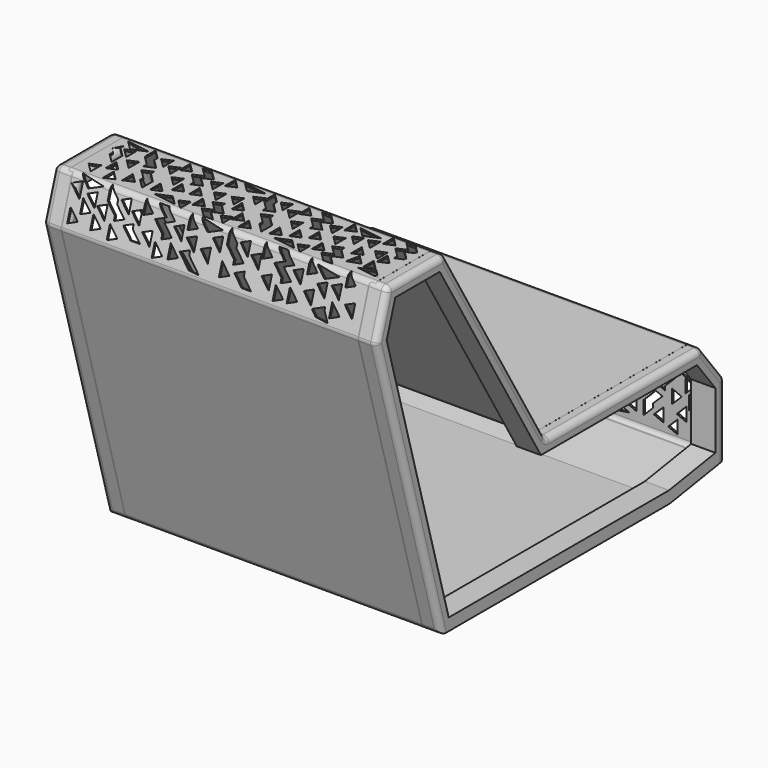
from build123d import *

# Parameters (mm, degrees)
F1_DEPTH  = 50.8
F2_R      = 12.7
F6_DEPTH  = 322.834
F9_DEPTH  = 25.4
F10_DEPTH = 25.4
F13_DEPTH = 25.4


with BuildPart() as f1:
    # F0 (on Right) → F1 (new body)
    with BuildSketch(Plane.YZ):
        Polygon((408.05088859, 0), (0, 0), (-265.7088614251, 447.3610464164), (-415.7088614251, 447.3610464164), (-446.1864444173, 352.1186349866), (-275.8783534847, -252.6389535836), (324.1216465153, -252.6389535836), (469.3139055241, -229.0369708183), (469.3139055241, -79.0369708183), align=None)
        Polygon((-256.6433629502, -227.2389464719), (-419.6670120859, 351.6518648302), (-397.1680678867, 421.9610393047), (-280.1650366436, 421.9610393047), (-14.4561752185, -25.4000071117), (395.6020354119, -25.4000071117), (443.9138984125, -87.7283660016), (443.9138984125, -207.4325008904), (322.0706361109, -227.2389464719), align=None, mode=Mode.SUBTRACT)
    extrude(amount=F1_DEPTH)

    # F2
    f2_edges = [f1.edges().sort_by_distance(p)[0] for p in [
        (25.4, -265.708861, 447.361046),
        (25.4, -415.708861, 447.361046),
        (0, -340.708861, 447.361046),
        (50.8, -340.708861, 447.361046),
        (25.4, 0, 0),
        (0, -132.854431, 223.680523),
        (50.8, -132.854431, 223.680523),
        (25.4, 408.050889, 0),
        (0, 204.025444, 0),
        (50.8, 204.025444, 0),
        (25.4, 469.313906, -79.036971),
        (0, 438.682397, -39.518485),
        (50.8, 438.682397, -39.518485),
        (25.4, 469.313906, -229.036971),
        (0, 469.313906, -154.036971),
        (50.8, 469.313906, -154.036971),
        (25.4, -446.186444, 352.118635),
        (25.4, -275.878353, -252.638954),
        (0, -361.032399, 49.739841),
        (50.8, -361.032399, 49.739841),
        (0, -430.947653, 399.739841),
        (50.8, -430.947653, 399.739841),
    ]]
    fillet(f2_edges, radius=F2_R)


with BuildPart() as f4_1:
    # F4: instance of F1
    add(f1.part.mirror(Plane.YZ.offset(-300)))


with BuildPart() as f6:
    # F5 (on offset) → F6 (new body, symmetric)
    with BuildSketch(Plane.YZ.offset(-300)):
        with BuildLine():
            Line((-272.8356088733, 447.4316021146), (-406.3371291142, 447.4316021146))
            ThreePointArc((-406.3371291142, 447.4316021146), (-413.8248759846, 444.9894599223), (-418.4329153658, 438.6022551546))
            Line((-418.4329153658, 438.6022551546), (-444.9211800784, 355.8264587119))
            ThreePointArc((-444.9211800784, 355.8264587119), (-445.5234270705, 352.1793045345), (-445.0499009192, 348.513215608))
            Line((-445.0499009192, 348.513215608), (-278.3840298653, -243.3109879494))
            ThreePointArc((-278.3840298653, -243.3109879494), (-273.8266312953, -249.992895251), (-266.1595227729, -252.5683978854))
            Line((-266.1595227729, -252.5683978854), (-262.5830273378, -252.5683978854))
            Line((-262.5830273378, -252.5683978854), (324.2229846526, -252.5683978854))
            Line((324.2229846526, -252.5683978854), (456.7152436615, -231.0308859339))
            Line((456.7152436615, -231.0308859339), (458.7529669103, -230.699640251))
            ThreePointArc((458.7529669103, -230.699640251), (466.3891540719, -226.3925157803), (469.4152436615, -218.1641831807))
            Line((469.4152436615, -218.1641831807), (469.4152436615, -83.312111495))
            ThreePointArc((469.4152436615, -83.312111495), (468.7312482019, -79.2004652452), (466.7529389554, -75.5317083444))
            Line((466.7529389554, -75.5317083444), (411.9654971749, -4.8490411512))
            ThreePointArc((411.9654971749, -4.8490411512), (407.5170272293, -1.2254730634), (401.927801881, 0.0705556982))
            Line((401.927801881, 0.0705556982), (7.3294237228, 0.0705556982))
            ThreePointArc((7.3294237228, 0.0705556982), (1.0475059475, 1.7330057407), (-3.5897859266, 6.2851211999))
            Line((-3.5897859266, 6.2851211999), (-261.9163992238, 441.2170366128))
            ThreePointArc((-261.9163992238, 441.2170366128), (-266.5536910979, 445.769152072), (-272.8356088733, 447.4316021146))
        make_face()
        with BuildLine():
            ThreePointArc((-414.8041674125, 437.4410553777), (-411.5785444469, 441.9120923374), (-406.3371291142, 443.6215894334))
            Line((-406.3371291142, 443.6215894334), (-272.8356088733, 443.6215894334))
            ThreePointArc((-272.8356088733, 443.6215894334), (-268.4382727031, 442.4578760637), (-265.1921730216, 439.2713997876))
            Line((-265.1921730216, 439.2713997876), (-6.8655597245, 4.3394843746))
            ThreePointArc((-6.8655597245, 4.3394843746), (-0.8370756577, -1.5782702677), (7.3294237228, -3.739456983))
            Line((7.3294237228, -3.739456983), (401.927801881, -3.739456983))
            ThreePointArc((401.927801881, -3.739456983), (405.8402540439, -4.646675822), (408.954178564, -7.1831698652))
            Line((408.954178564, -7.1831698652), (463.7416203444, -77.8658370584))
            ThreePointArc((463.7416203444, -77.8658370584), (465.1264348416, -80.4339632257), (465.6052309803, -83.312111495))
            Line((465.6052309803, -83.312111495), (465.6052309803, -218.1641831807))
            ThreePointArc((465.6052309803, -218.1641831807), (463.4869712893, -223.9240077843), (458.1416479009, -226.938990613))
            Line((458.1416479009, -226.938990613), (456.1039246521, -227.270236296))
            Line((456.1039246521, -227.270236296), (323.9153321541, -248.7583852043))
            Line((323.9153321541, -248.7583852043), (-262.5830273378, -248.7583852043))
            Line((-262.5830273378, -248.7583852043), (-266.1595227729, -248.7583852043))
            ThreePointArc((-266.1595227729, -248.7583852043), (-271.5264910828, -246.9555359319), (-274.7166655312, -242.2782074927))
            Line((-274.7166655312, -242.2782074927), (-441.3825365851, 349.5459960647))
            ThreePointArc((-441.3825365851, 349.5459960647), (-441.7140044182, 352.1122546526), (-441.2924321251, 354.665258935))
            Line((-441.2924321251, 354.665258935), (-414.8041674125, 437.4410553777))
        make_face(mode=Mode.SUBTRACT)
    extrude(amount=F6_DEPTH, both=True)

    # F8 (on face) → F9 (cut)
    with BuildSketch(Plane(origin=(0, -506.8810328427, 162.2019908326), x_dir=(1, 0, 0), z_dir=(0, -0.9524241143, 0.3047758299))):
        Polygon((-610.2134572743, 280.1658902577), (-587.9954886436, 258.1666408395), (-587.9954886436, 289.7434858457), align=None)
        Polygon((-553.3538012807, 290.2071253475), (-584.2335065195, 290.2071253475), (-575.091958046, 281.1555685521), align=None)
        Polygon((-545.7693254662, 293.3652272206), (-595.091958046, 300.9586835748), (-584.2335065195, 290.2071253475), (-553.3538012807, 290.2071253475), align=None)
        Polygon((-574.9599039268, 272.0962909685), (-554.9599039268, 252.2931759458), (-554.9599039268, 280.7177772503), align=None)
        Polygon((-561.2534010124, 243.4772804856), (-581.2534010124, 263.2803955084), (-581.2534010124, 234.8557942038), align=None)
        Polygon((-602.6199054718, 241.1658143859), (-602.6199054718, 212.7412130814), (-582.6199054718, 221.3626993632), align=None)
        Polygon((-554.9599039268, 243.671689664), (-554.9599039268, 215.2470883594), (-534.9599039268, 223.8685746412), align=None)
        Polygon((-550.9002315712, 258.1129518972), (-530.9002315712, 238.3098368745), (-530.9002315712, 266.734438179), align=None)
        Polygon((-521.3424320719, 290.2071253475), (-532.2008835983, 290.2071253475), (-532.2008835983, 272.5340822703), (-512.2008835983, 252.7309672475), (-512.2008835983, 244.1094809657), (-492.2008835983, 252.7309672475), (-512.2008835983, 272.5340822703), (-512.2008835983, 281.1555685521), align=None)
        Polygon((-532.2008835983, 300.9586835748), (-532.2008835983, 290.2071253475), (-521.3424320719, 290.2071253475), align=None)
        Polygon((-485.7396268845, 290.2071253475), (-487.70695417, 290.2071253475), (-505.7396268845, 282.4337033258), (-485.7396268845, 262.6305883031), align=None)
        Polygon((-498.8226485252, 217.7414104819), (-518.8226485252, 237.5445255047), (-518.8226485252, 209.1199242001), align=None)
        Polygon((-472.2404265404, 222.5241366963), (-452.2404265404, 222.5241366963), (-472.2404265404, 242.3272517191), (-472.2404265404, 250.9487380009), (-492.2404265404, 242.3272517191), align=None)
        Polygon((-480.7777786255, 270.2546862589), (-460.7777786255, 250.4515712361), (-460.7777786255, 278.8761725407), align=None)
        Polygon((-449.0202209381, 290.2071253475), (-458.018758297, 290.2071253475), (-458.018758297, 270.6924775606), (-438.018758297, 279.3139638424), align=None)
        Polygon((-458.018758297, 299.1170788652), (-458.018758297, 290.2071253475), (-449.0202209381, 290.2071253475), align=None)
        Polygon((-431.9680453543, 299.385476847), (-422.6984415682, 290.2071253475), (-403.0085313252, 290.2071253475), (-412.2482537937, 299.3558896886), align=None)
        Polygon((-403.0085313252, 290.2071253475), (-422.6984415682, 290.2071253475), (-412.3803079128, 279.9905659676), (-432.3803079128, 271.3690796858), (-412.3803079128, 251.5659646631), (-412.2482537937, 242.5066870795), (-392.2482537937, 251.1281733613), (-412.2482537937, 270.9312883841), (-392.2482537937, 279.5527746659), align=None)
        Polygon((-432.3803079128, 223.1413633585), (-432.3803079128, 251.5659646631), (-452.3803079128, 242.9444783813), align=None)
        Polygon((-403.8098454475, 215.9172997356), (-423.8098454475, 235.7204147583), (-423.8098454475, 207.2958134538), align=None)
        Polygon((-392.2482537937, 242.5066870795), (-392.2482537937, 214.082085775), (-372.2482537937, 222.7035720568), align=None)
        Polygon((-392.2482537937, 270.9312883841), (-372.2482537937, 251.1281733613), (-372.2482537937, 279.5527746659), align=None)
        Polygon((-353.3391356283, 290.2071253475), (-364.628246994, 290.2071253475), (-364.628246994, 272.9605025869), (-344.628246994, 281.5819888687), align=None)
        Polygon((-364.628246994, 301.3851038914), (-364.628246994, 290.2071253475), (-353.3391356283, 290.2071253475), align=None)
        Polygon((-344.628246994, 301.3851038914), (-333.3391356283, 290.2071253475), (-303.9141783387, 290.2071253475), (-295.3056144142, 293.7916475372), align=None)
        Polygon((-303.9141783387, 290.2071253475), (-333.3391356283, 290.2071253475), (-324.628246994, 281.5819888687), align=None)
        Polygon((-343.1586944771, 240.5479399776), (-343.1586944771, 268.9725412821), (-363.1586944771, 260.3510550003), align=None)
        Polygon((-351.315243187, 233.4173643909), (-351.4472973061, 242.4766419744), (-371.4472973061, 233.8551556926), (-346.7147119375, 209.3660440495), (-324.8525857925, 207.1910202503), align=None)
        Polygon((-331.7133914852, 250.4200275026), (-311.7133914852, 230.6169124798), (-311.7133914852, 259.0415137844), align=None)
        Polygon((-312.1250509644, 275.4354114614), (-292.1250509644, 255.6322964386), (-292.1250509644, 284.0568977432), align=None)
        Polygon((-270.4480611807, 290.2071253475), (-281.7371725464, 290.2071253475), (-281.7371725464, 272.9605025869), (-261.7371725464, 253.1573875641), (-261.7371725464, 244.5359012824), (-241.7371725464, 253.1573875641), (-261.7371725464, 272.9605025869), (-261.7371725464, 281.5819888687), align=None)
        Polygon((-281.7371725464, 301.3851038914), (-281.7371725464, 290.2071253475), (-270.4480611807, 290.2071253475), align=None)
        Polygon((-284.7306370163, 244.4622198544), (-284.7306370163, 216.0376185498), (-264.7306370163, 224.6591048316), align=None)
        Polygon((-236.1780321312, 212.2973443464), (-216.1780321312, 212.2973443464), (-236.1780321312, 232.1004593692), (-236.1780321312, 240.721945651), (-256.1780321312, 232.1004593692), align=None)
        Polygon((-236.1780619335, 264.8613008217), (-236.1780619335, 290.2071253475), (-243.3201640681, 290.2071253475), (-256.1780619335, 284.6644158445), align=None)
        Polygon((-243.3201640681, 290.2071253475), (-236.1780619335, 290.2071253475), (-236.1780619335, 293.2859021263), align=None)
        Polygon((-207.555047245, 290.2071253475), (-198.1258500469, 290.2071253475), (-207.555047245, 299.5434991818), align=None)
        Polygon((-187.555047245, 279.7403841591), (-198.1258500469, 290.2071253475), (-207.555047245, 290.2071253475), (-207.555047245, 271.1188978773), align=None)
        Polygon((-230.3140675735, 270.6811065755), (-210.3140675735, 250.8779915528), (-210.3140675735, 279.3025928573), align=None)
        Polygon((-181.9165968609, 223.5677836751), (-181.9165968609, 251.9923849797), (-201.9165968609, 243.3708986979), align=None)
        Polygon((-150.3972542, 218.5057593321), (-170.3972542, 238.3088743549), (-170.3972542, 209.8842730503), align=None)
        Polygon((-141.7845427418, 279.9791949825), (-152.114160434, 290.2071253475), (-171.804070677, 290.2071253475), (-161.9165968609, 280.4169862842), (-181.9165968609, 271.7955000024), (-161.9165968609, 251.9923849797), (-161.7845427418, 242.9331073961), (-141.7845427418, 251.5545936779), (-161.7845427418, 271.3577087007), align=None)
        Polygon((-171.804070677, 290.2071253475), (-152.114160434, 290.2071253475), (-161.7845427418, 299.7823100052), (-181.5043343023, 299.8118971637), align=None)
        Polygon((-113.2840113342, 290.2071253475), (-102.2302799566, 290.2071253475), (-113.2840113342, 301.1520410425), align=None)
        Polygon((-93.2840113342, 281.3489260197), (-102.2302799566, 290.2071253475), (-113.2840113342, 290.2071253475), (-113.2840113342, 272.7274397379), align=None)
        Polygon((-141.7845427418, 271.3577087007), (-121.7845427418, 251.5545936779), (-121.7845427418, 279.9791949825), align=None)
        Polygon((-93.2840113342, 224.4997234106), (-93.2840113342, 252.9243247152), (-113.2840113342, 244.3028384334), align=None)
        Polygon((-141.7845427418, 242.9331073961), (-141.7845427418, 214.5085060916), (-121.7845427418, 223.1299923734), align=None)
        Polygon((-64.8736751787, 225.3813321149), (-64.9616606534, 231.4173788786), (-90.336183123, 220.4790740097), (-80.0273045897, 209.706902504), (-54.0199615061, 206.7942172289), align=None)
        Polygon((-53.1519572151, 243.8650471316), (-53.1519572151, 215.4404458271), (-33.1519572151, 224.0619321089), align=None)
        Polygon((-7.5135068309, 226.7677186346), (-7.5135068309, 255.1923199391), (-27.5135068309, 246.5708336573), align=None)
        Polygon((-60.820243777, 269.5832101332), (-40.820243777, 249.7800951104), (-40.820243777, 278.204696415), align=None)
        Polygon((-89.8417569411, 263.7192157732), (-69.8417569411, 243.9161007505), (-69.8417569411, 272.340702055), align=None)
        Polygon((-48.0119017971, 287.9891266804), (-62.4187184316, 290.2071253475), (-91.9056332358, 290.2071253475), (-77.3345343769, 275.7794680119), align=None)
        Polygon((-91.9056332358, 290.2071253475), (-62.4187184316, 290.2071253475), (-97.3345343769, 295.5825830346), align=None)
        Polygon((-33.1519572151, 290.2071253475), (-20.4910109151, 290.2071253475), (-33.1519572151, 302.7434341412), align=None)
        Polygon((-13.1519572151, 282.9403191185), (-20.4910109151, 290.2071253475), (-33.1519572151, 290.2071253475), (-33.1519572151, 274.3188328367), align=None)
    extrude(amount=-F9_DEPTH, mode=Mode.SUBTRACT)

    # F7 (on face) → F10 (cut)
    with BuildSketch(Plane.XY.offset(447.4316021146)):
        Polygon((-558.2723617554, -283.5318148136), (-607.5949943352, -275.9383584594), (-587.5949943352, -295.7414734821), align=None)
        Polygon((-602.6913714409, -330.5999256248), (-582.6913714409, -350.4030406475), (-582.6913714409, -321.978439343), (-602.6913714409, -302.1753243202), (-602.6913714409, -293.5538380384), (-612.6913714409, -312.0768818316), (-602.6913714409, -321.978439343), align=None)
        Polygon((-595.1479458809, -301.6980014795), (-575.1479458809, -321.5011165023), (-575.1479458809, -293.0765151978), align=None)
        Polygon((-608.7343287468, -378.1811335678), (-588.7343287468, -397.9842485905), (-588.7343287468, -369.559647286), align=None)
        Polygon((-576.9602847099, -344.9864812726), (-576.9602847099, -373.4110825772), (-556.9602847099, -364.7895962954), align=None)
        Polygon((-538.9182567596, -394.1856687169), (-558.9182567596, -374.3825536942), (-558.9182567596, -402.8071549987), align=None)
        Polygon((-567.4963188171, -329.8447750563), (-547.4963188171, -349.647890079), (-547.4963188171, -321.2232887745), align=None)
        Polygon((-532.3889255524, -292.638723896), (-552.3889255524, -272.8356088733), (-552.3889255524, -301.2602101778), (-532.3889255524, -321.0633252005), (-532.3889255524, -329.6848114823), (-512.3889255524, -321.0633252005), (-532.3889255524, -301.2602101778), align=None)
        Polygon((-525.9276688385, -291.3605891222), (-505.9276688385, -311.163704145), (-505.9276688385, -282.7391028404), align=None)
        Polygon((-500.9658205795, -303.5396061892), (-480.9658205795, -323.3427212119), (-480.9658205795, -294.9181199074), align=None)
        Polygon((-506.8297851372, -370.5448547), (-486.8297851372, -390.3479697228), (-486.8297851372, -361.9233684183), (-506.8297851372, -342.1202533955), (-506.8297851372, -333.4987671137), (-526.8297851372, -342.1202533955), (-506.8297851372, -361.9233684183), align=None)
        Polygon((-508.7803411484, -381.5211420159), (-528.7803411484, -361.7180269932), (-528.7803411484, -390.1426282977), align=None)
        Polygon((-452.5683498669, -350.6529290895), (-452.5683498669, -322.228327785), (-472.5683498669, -330.8498140668), align=None)
        Polygon((-452.5683498669, -379.0775303941), (-472.5683498669, -359.2744153713), (-472.5683498669, -387.6990166759), align=None)
        Polygon((-458.206800251, -294.4803286056), (-478.206800251, -274.6772135829), (-478.206800251, -303.1018148874), align=None)
        Polygon((-432.5683498669, -322.228327785), (-432.4362957478, -331.2876053685), (-412.4362957478, -322.6661190868), (-432.4362957478, -302.863004064), (-412.4362957478, -294.2415177822), (-432.4362957478, -274.4384027595), (-452.1560873083, -274.408815601), (-432.5683498669, -293.8037264805), (-452.5683498669, -302.4252127623), align=None)
        Polygon((-423.9978874016, -357.8769927125), (-443.9978874016, -338.0738776898), (-443.9978874016, -366.4984789943), align=None)
        Polygon((-457.7084052849, -394.7770086383), (-408.3857727051, -402.3704649926), (-428.3857727051, -382.5673499698), align=None)
        Polygon((-412.4362957478, -388.1368079776), (-394.0550248057, -406.3371291142), (-392.4362957478, -406.3371291142), (-392.4362957478, -379.5153216958), align=None)
        Polygon((-412.4362957478, -331.2876053685), (-412.4362957478, -359.7122066731), (-392.4362957478, -351.0907203913), align=None)
        Polygon((-412.4362957478, -302.863004064), (-392.4362957478, -322.6661190868), (-392.4362957478, -294.2415177822), align=None)
        Polygon((-384.3856291088, -272.8356088733), (-384.8162889481, -272.8356088733), (-384.8162889481, -300.8337898612), (-364.8162889481, -292.2123035794), align=None)
        Polygon((-364.8162889481, -349.0615061885), (-364.8162889481, -320.6369048839), (-384.8162889481, -329.2583911657), align=None)
        Polygon((-364.8162889481, -377.486107493), (-384.8162889481, -357.6829924703), (-384.8162889481, -386.1075937748), align=None)
        Polygon((-344.6842348289, -358.120783772), (-344.8162889481, -349.0615061885), (-364.8162889481, -357.6829924703), (-344.8162889481, -377.486107493), (-364.8162889481, -386.1075937748), (-344.8162889481, -405.9107087975), (-325.0964973875, -405.940295956), (-344.6842348289, -386.5453850765), (-324.6842348289, -377.9238987948), align=None)
        Polygon((-362.0465130225, -272.8356088733), (-364.3856291088, -272.8356088733), (-344.8162889481, -292.2123035794), (-315.4936563683, -280.0026449109), align=None)
        Polygon((-324.6842348289, -301.2715811629), (-304.6842348289, -321.0746961857), (-304.6842348289, -292.6500948811), align=None)
        Polygon((-324.6842348289, -329.6961824675), (-324.6842348289, -358.120783772), (-304.6842348289, -349.4992974902), align=None)
        Polygon((-324.6842348289, -386.5453850765), (-304.6957188658, -406.3371291142), (-304.6842348289, -406.3371291142), (-304.6842348289, -377.9238987948), align=None)
        Polygon((-281.9252145004, -377.486107493), (-301.9252145004, -357.6829924703), (-301.9252145004, -386.1075937748), align=None)
        Polygon((-256.9633960438, -391.4694465643), (-276.9633960438, -371.6663315415), (-276.9633960438, -400.0909328461), align=None)
        Polygon((-256.3660740852, -370.1184343834), (-236.3660740852, -389.9215494062), (-236.3660740852, -361.4969481016), (-256.3660740852, -341.6938330789), (-256.3660740852, -333.0723467971), (-276.3660740852, -341.6938330789), (-256.3660740852, -361.4969481016), align=None)
        Polygon((-301.4945546612, -272.8356088733), (-301.9252145004, -272.8356088733), (-301.9252145004, -300.8337898612), (-281.9252145004, -320.6369048839), (-281.9252145004, -329.2583911657), (-261.9252145004, -320.6369048839), (-281.9252145004, -300.8337898612), (-281.9252145004, -292.2123035794), align=None)
        Polygon((-276.3661038876, -289.1298766036), (-256.3661038876, -308.9329916263), (-256.3661038876, -280.5083903218), align=None)
        Polygon((-250.5021095276, -303.1131858725), (-230.5021095276, -322.9163008953), (-230.5021095276, -294.4916995908), align=None)
        Polygon((-207.7430891991, -294.053908289), (-227.7430891991, -274.2507932663), (-227.7430891991, -302.6753945708), align=None)
        Polygon((-202.1046388149, -350.2265087729), (-202.1046388149, -321.8019074684), (-222.1046388149, -330.4233937502), align=None)
        Polygon((-202.1046388149, -378.6511100775), (-222.1046388149, -358.8479950547), (-222.1046388149, -387.2725963593), align=None)
        Polygon((-171.2788259983, -365.1188589578), (-191.2788259983, -345.3157439351), (-191.2788259983, -373.7403452396), align=None)
        Polygon((-207.2446942329, -394.3505883217), (-157.9220616531, -401.9440446759), (-177.9220616531, -382.1409296532), align=None)
        Polygon((-182.1046388149, -321.8019074684), (-181.9725846958, -330.8611850519), (-161.9725846958, -322.2396987701), (-181.9725846958, -302.4365837474), (-161.9725846958, -293.8150974656), (-181.9725846958, -274.0119824428), (-201.6923762564, -273.9823952844), (-182.1046388149, -293.3773061638), (-202.1046388149, -301.9987924456), align=None)
        Polygon((-161.9725846958, -302.4365837474), (-141.9725846958, -322.2396987701), (-141.9725846958, -293.8150974656), align=None)
        Polygon((-133.2767734371, -272.8356088733), (-133.4720532882, -272.8356088733), (-133.4720532882, -301.0668527101), (-113.4720532882, -292.4453664284), align=None)
        Polygon((-113.4720532882, -349.2945690374), (-113.4720532882, -320.8699677329), (-133.4720532882, -329.4914540147), align=None)
        Polygon((-113.4720532882, -377.719170342), (-133.4720532882, -357.9160553192), (-133.4720532882, -386.3406566238), align=None)
        Polygon((-93.3399991691, -358.353846621), (-93.4720532882, -349.2945690374), (-113.4720532882, -357.9160553192), (-93.4720532882, -377.719170342), (-113.4720532882, -386.3406566238), (-93.4720532882, -406.1437716465), (-73.7522617277, -406.1733588049), (-93.3399991691, -386.7784479255), (-73.3399991691, -378.1569616437), align=None)
        Polygon((-110.0297988951, -310.0750766749), (-90.0297988951, -329.8781916976), (-90.0297988951, -301.4535903931), align=None)
        Polygon((-68.1999437511, -285.8051657677), (-117.5225763309, -278.2117094134), (-97.5225763309, -298.0148244362), align=None)
        Polygon((-81.0082857311, -304.2110823149), (-61.0082857311, -324.0141973376), (-61.0082857311, -295.5895960331), align=None)
        Polygon((-73.3399991691, -329.9292453164), (-73.3399991691, -358.353846621), (-53.3399991691, -349.7323603392), align=None)
        Polygon((-36.2719590962, -376.353321219), (-56.2719590962, -356.5502061963), (-62.1359534562, -384.9748075008), align=None)
        Polygon((-7.701548785, -375.451175118), (-27.701548785, -355.6480600953), (-27.701548785, -384.0726613998), align=None)
        Polygon((-32.841604203, -391.1506533623), (16.4810283768, -398.7441097165), (-3.5189716232, -378.9409946938), align=None)
        Polygon((-21.7614667763, -326.5162448664), (-21.7614667763, -354.9408461709), (-1.7614667763, -346.3193598891), align=None)
        Polygon((-27.701548785, -347.0265738135), (-27.701548785, -318.601972509), (-47.701548785, -327.2234587908), align=None)
        Polygon((-51.5375043956, -272.8356088733), (-53.3399991691, -272.8356088733), (-53.3399991691, -299.4754596114), (-33.3399991691, -290.8539733296), align=None)
        Polygon((12.4305053341, -290.6151625062), (-5.5258147827, -272.8356088733), (-25.2157250257, -272.8356088733), (-7.701548785, -290.1773712044), (-27.701548785, -298.7988574862), (-7.701548785, -318.601972509), (-7.5694946659, -327.6612500925), (12.4305053341, -319.0397638107), (-7.5694946659, -299.236648788), align=None)
        Polygon((-351.9014334393, -323.3742649455), (-331.9014334393, -343.1773799682), (-331.9014334393, -314.7527786637), align=None)
        Polygon((-161.9725846958, -330.8611850519), (-161.9725846958, -359.2857863565), (-141.9725846958, -350.6643000747), align=None)
        Polygon((-161.9725846958, -387.710387661), (-143.1606539145, -406.3371291142), (-141.9725846958, -406.3371291142), (-141.9725846958, -379.0889013792), align=None)
    extrude(amount=-F10_DEPTH, mode=Mode.SUBTRACT)

    # F11 (on face) + F12 (on face) → F13 (cut)
    with BuildSketch(Plane(origin=(0, 469.4152436615, 0), x_dir=(-1, 0, 0), z_dir=(0, 1, 0))):
        Polygon((46.4639700949, -94.8217539072), (-2.8586624849, -87.2282975529), (17.1413375151, -107.0314125757), align=None)
        Polygon((9.5883859694, -112.9879405731), (29.5883859694, -132.7910555958), (29.5883859694, -104.3664542913), align=None)
        Polygon((2.0449604094, -141.8898647183), (22.0449604094, -161.6929797411), (22.0449604094, -133.2683784365), (2.0449604094, -113.4652634138), (2.0449604094, -104.843777132), (-7.9550395906, -123.3668209251), (2.0449604094, -133.2683784365), align=None)
        Polygon((37.2400130332, -141.1347141498), (57.2400130332, -160.9378291726), (57.2400130332, -132.513227868), align=None)
        Polygon((27.7760471404, -156.2764203662), (27.7760471404, -184.7010216707), (47.7760471404, -176.0795353889), align=None)
        Polygon((-3.9979968965, -189.4710726613), (16.0020031035, -209.2741876841), (16.0020031035, -180.8495863795), align=None)
        Polygon((65.8180750906, -205.4756078105), (45.8180750906, -185.6724927877), (45.8180750906, -214.0970940923), align=None)
        Polygon((95.9559907019, -192.8110811095), (75.9559907019, -173.0079660867), (75.9559907019, -201.4325673913), align=None)
        Polygon((97.9065467131, -181.8347937936), (117.9065467131, -201.6379088163), (117.9065467131, -173.2133075118), (97.9065467131, -153.410192489), (97.9065467131, -144.7887062073), (77.9065467131, -153.410192489), (97.9065467131, -173.2133075118), align=None)
        Polygon((78.8086630118, -102.6505282158), (98.8086630118, -122.4536432385), (98.8086630118, -94.029041934), align=None)
        Polygon((103.7705112708, -114.8295452827), (123.7705112708, -134.6326603055), (123.7705112708, -106.2080590009), align=None)
        Polygon((146.5295315993, -105.7702676992), (126.5295315993, -85.9671526764), (126.5295315993, -114.391753981), align=None)
        Polygon((152.1679819834, -161.9428681831), (152.1679819834, -133.5182668785), (132.1679819834, -142.1397531603), align=None)
        Polygon((152.1679819834, -190.3674694876), (132.1679819834, -170.5643544649), (132.1679819834, -198.9889557694), align=None)
        Polygon((180.7384444487, -169.1669318061), (160.7384444487, -149.3638167833), (160.7384444487, -177.7884180878), align=None)
        Polygon((147.0279265654, -206.0669477319), (196.3505591452, -213.6604040861), (176.3505591452, -193.8572890634), align=None)
        Polygon((192.3000361025, -199.4267470712), (211.2237620799, -218.1641831807), (212.3000361025, -218.1641831807), (212.3000361025, -190.8052607894), align=None)
        Polygon((192.3000361025, -142.5775444621), (192.3000361025, -171.0021457666), (212.3000361025, -162.3806594848), align=None)
        Polygon((172.1679819834, -133.5182668785), (172.3000361025, -142.5775444621), (192.3000361025, -133.9560581803), (172.3000361025, -114.1529431576), (192.3000361025, -105.5314568758), (172.3000361025, -85.728341853), (152.580244542, -85.6987546946), (172.1679819834, -105.093665574), (152.1679819834, -113.7151518558), align=None)
        Polygon((192.3000361025, -114.1529431576), (212.3000361025, -133.9560581803), (212.3000361025, -105.5314568758), align=None)
        Polygon((239.9200429022, -103.5022426729), (219.9200429022, -83.6991276502), (219.9200429022, -112.1237289547), align=None)
        Polygon((239.9200429022, -160.351445282), (239.9200429022, -131.9268439775), (219.9200429022, -140.5483302593), align=None)
        Polygon((239.9200429022, -188.7760465865), (219.9200429022, -168.9729315638), (219.9200429022, -197.3975328683), align=None)
        Polygon((260.0520970213, -169.4107228655), (259.9200429022, -160.351445282), (239.9200429022, -168.9729315638), (259.9200429022, -188.7760465865), (239.9200429022, -197.3975328683), (259.9200429022, -217.2006478911), (279.6398344628, -217.2302350495), (260.0520970213, -197.8353241701), (280.0520970213, -189.2138378883), align=None)
        Polygon((252.834898411, -134.664204039), (272.834898411, -154.4673190618), (272.834898411, -126.0427177572), align=None)
        Polygon((280.0520970213, -140.986121561), (280.0520970213, -169.4107228655), (300.0520970213, -160.7892365838), align=None)
        Polygon((280.0520970213, -112.5615202565), (300.0520970213, -132.3646352792), (300.0520970213, -103.9400339747), align=None)
        Polygon((289.242675482, -91.2925840044), (239.9200429022, -83.6991276502), (259.9200429022, -103.5022426729), align=None)
        Polygon((322.8111173499, -103.5022426729), (302.8111173499, -83.6991276502), (302.8111173499, -112.1237289547), (322.8111173499, -131.9268439775), (322.8111173499, -140.5483302593), (342.8111173499, -131.9268439775), (322.8111173499, -112.1237289547), align=None)
        Polygon((328.3702279627, -100.4198156971), (348.3702279627, -120.2229307199), (348.3702279627, -91.7983294153), align=None)
        Polygon((354.2342223227, -114.4031249661), (374.2342223227, -134.2062399888), (374.2342223227, -105.7816386843), align=None)
        Polygon((348.3702577651, -181.408373477), (368.3702577651, -201.2114884997), (368.3702577651, -172.7868871952), (348.3702577651, -152.9837721724), (348.3702577651, -144.3622858906), (328.3702577651, -152.9837721724), (348.3702577651, -172.7868871952), align=None)
        Polygon((347.7729358065, -202.7593856578), (327.7729358065, -182.9562706351), (327.7729358065, -211.3808719396), align=None)
        Polygon((322.8111173499, -188.7760465865), (302.8111173499, -168.9729315638), (302.8111173499, -197.3975328683), align=None)
        Polygon((280.0520970213, -197.8353241701), (300.0520970213, -217.6384391928), (300.0520970213, -189.2138378883), align=None)
        Polygon((402.6316930354, -189.941049171), (382.6316930354, -170.1379341483), (382.6316930354, -198.5625354528), align=None)
        Polygon((397.4916376173, -205.6405274152), (446.8142701972, -213.2339837695), (426.8142701972, -193.4308687467), align=None)
        Polygon((442.7637471545, -199.0003267545), (462.1181329711, -218.1641831807), (462.7637471545, -218.1641831807), (462.7637471545, -190.3788404728), align=None)
        Polygon((433.457505852, -176.4087980514), (413.457505852, -156.6056830286), (413.457505852, -185.0302843332), align=None)
        Polygon((402.6316930354, -161.5164478665), (402.6316930354, -133.0918465619), (382.6316930354, -141.7133328437), align=None)
        Polygon((396.9932426512, -105.3438473825), (376.9932426512, -85.5407323598), (376.9932426512, -113.9653336643), align=None)
        Polygon((422.6316930354, -133.0918465619), (422.7637471545, -142.1511241455), (442.7637471545, -133.5296378637), (422.7637471545, -113.7265228409), (442.7637471545, -105.1050365591), (422.7637471545, -85.3019215364), (403.0439555939, -85.272334378), (422.6316930354, -104.6672452574), (402.6316930354, -113.2887315392), align=None)
        Polygon((491.2642785621, -103.7353055219), (471.2642785621, -83.9321904991), (471.2642785621, -112.3567918037), align=None)
        Polygon((491.2642785621, -160.584508131), (491.2642785621, -132.1599068264), (471.2642785621, -140.7813931082), align=None)
        Polygon((442.7637471545, -142.1511241455), (442.7637471545, -170.57572545), (462.7637471545, -161.9542391682), align=None)
        Polygon((491.2642785621, -189.0091094355), (471.2642785621, -169.2059944128), (471.2642785621, -197.6305957173), align=None)
        Polygon((511.3963326812, -169.6437857145), (511.2642785621, -160.584508131), (491.2642785621, -169.2059944128), (511.2642785621, -189.0091094355), (491.2642785621, -197.6305957173), (511.2642785621, -217.4337107401), (530.9840701226, -217.4632978985), (511.3963326812, -198.0683870191), (531.3963326812, -189.4469007373), align=None)
        Polygon((531.3963326812, -141.21918441), (531.3963326812, -169.6437857145), (551.3963326812, -161.0222994327), align=None)
        Polygon((568.4643727541, -187.6432603126), (548.4643727541, -167.8401452898), (542.6003783941, -196.2647465944), align=None)
        Polygon((536.5363880992, -97.0951048612), (487.2137555194, -89.501648507), (507.2137555194, -109.3047635297), align=None)
        Polygon((523.7280461192, -115.5010214084), (543.7280461192, -135.3041364312), (543.7280461192, -106.8795351266), align=None)
        Polygon((552.3773036986, -83.312111495), (551.3963326812, -83.312111495), (551.3963326812, -110.7653987049), (571.3963326812, -102.1439124231), align=None)
        Polygon((598.3889933116, -83.312111495), (578.6990830685, -83.312111495), (597.0347830653, -101.467310298), (577.0347830653, -110.0887965798), (597.0347830653, -129.8919116025), (597.1668371844, -138.9511891861), (617.1668371844, -130.3297029043), (597.1668371844, -110.5265878815), (617.1668371844, -101.9051015997), align=None)
        Polygon((577.0347830653, -158.316512907), (577.0347830653, -129.8919116025), (557.0347830653, -138.5133978843), align=None)
        Polygon((582.974865074, -137.8061839599), (582.974865074, -166.2307852645), (602.974865074, -157.6092989827), align=None)
        Polygon((597.0347830653, -186.7411142116), (577.0347830653, -166.9379991888), (577.0347830653, -195.3626004934), align=None)
        Polygon((571.8947276473, -202.4405924558), (621.2173602271, -210.0340488101), (601.2173602271, -190.2309337873), align=None)
        Polygon((72.3474062979, -103.9286629895), (52.3474062979, -84.1255479668), (52.3474062979, -112.5501492713), (72.3474062979, -132.3532642941), (72.3474062979, -140.9747505759), (92.3474062979, -132.3532642941), (72.3474062979, -112.5501492713), align=None)
        Polygon((442.7637471545, -113.7265228409), (462.7637471545, -133.5296378637), (462.7637471545, -105.1050365591), align=None)
        Polygon((494.7065329552, -121.3650157684), (514.7065329552, -141.1681307912), (514.7065329552, -112.7435294866), align=None)
    with BuildSketch(Plane(origin=(0, 255.0004414672, 197.655555395), x_dir=(-1, 0, 0), z_dir=(0, 0.7903697082, 0.6126301693))):
        Polygon((575.2227269113, -338.8113110873), (619.609747909, -345.6449063156), (622.834, -345.6449063156), (622.834, -344.7102549992), (604.5453594911, -326.6016524188), align=None)
        Polygon((600.3627823293, -323.1118328431), (580.3627823293, -303.3087178204), (580.3627823293, -331.7333191249), align=None)
        Polygon((586.302864338, -274.1769025914), (586.302864338, -302.601503896), (606.302864338, -293.9800176142), align=None)
        Polygon((580.3627823293, -294.6872315386), (580.3627823293, -266.262630234), (560.3627823293, -274.8841165158), align=None)
        Polygon((620.4948364484, -266.7004215358), (609.9051953875, -256.2150275368), (590.2152851445, -256.2150275368), (600.3627823293, -266.262630234), (600.4948364484, -275.3219078176), align=None)
        Polygon((547.0560453832, -271.6748550627), (547.0560453832, -256.2150275368), (531.4425143724, -256.2150275368), align=None)
        Polygon((534.7243319452, -277.5899030415), (534.7243319452, -306.014504346), (554.7243319452, -297.3930180642), align=None)
        Polygon((571.7923720181, -324.0139789441), (551.7923720181, -304.2108639214), (545.9283776581, -332.6354652259), align=None)
        Polygon((526.0415420428, -345.6449063156), (506.3516317998, -345.6449063156), (514.5922778261, -353.8044293716), (534.3120693866, -353.83401653), align=None)
        Polygon((494.5922778261, -334.0013143488), (506.3516317998, -345.6449063156), (526.0415420428, -345.6449063156), (514.7243319452, -334.4391056506), (534.7243319452, -325.8176193688), (514.7243319452, -306.014504346), (514.5922778261, -296.9552267625), (494.5922778261, -305.5767130443), (514.5922778261, -325.379828067), align=None)
        Polygon((446.0917464185, -335.3710453861), (456.4677513225, -345.6449063156), (466.0917464185, -345.6449063156), (466.0917464185, -326.7495591043), align=None)
        Polygon((466.0917464185, -345.6449063156), (456.4677513225, -345.6449063156), (466.0917464185, -355.1741604088), align=None)
        Polygon((494.5922778261, -325.379828067), (474.5922778261, -305.5767130443), (474.5922778261, -334.0013143488), align=None)
        Polygon((400.8196368814, -342.0112460467), (424.4217598143, -345.6449063156), (446.1431046016, -345.6449063156), (430.1422694612, -329.8015873782), align=None)
        Polygon((446.1431046016, -345.6449063156), (424.4217598143, -345.6449063156), (450.1422694612, -349.604702401), align=None)
        Polygon((331.1009350705, -319.3269892666), (331.1009350705, -345.6449063156), (335.987990937, -345.6449063156), (351.1009350705, -339.1301042893), align=None)
        Polygon((283.3800962853, -334.2060428016), (294.9326863711, -345.6449063156), (303.3800962853, -345.6449063156), (303.3800962853, -325.5845565198), align=None)
        Polygon((243.2480421662, -333.7682514999), (255.2427761281, -345.6449063156), (274.9326863711, -345.6449063156), (263.3800962853, -334.2060428016), (283.3800962853, -325.5845565198), (263.3800962853, -305.7814414971), (263.2480421662, -296.7221639135), (243.2480421662, -305.3436501953), (263.2480421662, -325.1467652181), align=None)
        Polygon((195.6280353665, -335.7974657027), (205.5733804313, -345.6449063156), (215.6280353665, -345.6449063156), (215.6280353665, -327.1759794209), align=None)
        Polygon((150.3559258294, -342.4376663634), (171.1882728368, -345.6449063156), (195.2487337104, -345.6449063156), (179.6785584092, -330.2280076949), align=None)
        Polygon((243.2480421662, -325.1467652181), (223.2480421662, -305.3436501953), (223.2480421662, -333.7682514999), align=None)
        Polygon((155.4959812474, -326.7381881191), (135.4959812474, -306.9350730964), (135.4959812474, -335.3596744009), align=None)
        Polygon((101.2345459771, -318.2055124251), (121.2345459771, -338.0086274478), (121.2345459771, -309.5840261433), (101.2345459771, -289.7809111206), (101.2345459771, -281.1594248388), (81.2345459771, -289.7809111206), (101.2345459771, -309.5840261433), align=None)
        Polygon((99.2839899659, -329.181799741), (79.2839899659, -309.3786847183), (79.2839899659, -337.8032860228), align=None)
        Polygon((49.1460743546, -322.0432114192), (49.1460743546, -345.6449063156), (60.3341833432, -345.6449063156), (69.1460743546, -341.846326442), align=None)
        Polygon((-0.6699976325, -325.8417912928), (19.3300023675, -345.6449063156), (19.3300023675, -317.220305011), align=None)
        Polygon((31.1040464044, -292.6471389977), (31.1040464044, -321.0717403022), (51.1040464044, -312.4502540204), align=None)
        Polygon((11.8154264108, -256.2150275368), (-2.7253485425, -256.2150275368), (-4.6270403266, -259.7375395566), (5.3729596734, -269.639097068), (5.3729596734, -278.2605833498), (25.3729596734, -298.0636983726), (25.3729596734, -269.639097068), align=None)
        Polygon((40.5680122972, -277.5054327813), (60.5680122972, -297.3085478041), (60.5680122972, -268.8839464995), align=None)
        Polygon((32.9163852334, -256.2150275368), (19.8409204132, -256.2150275368), (32.9163852334, -269.1617742274), align=None)
        Polygon((83.0420846178, -256.2150275368), (63.0420846178, -256.2150275368), (75.6754055619, -268.7239829256), (75.6754055619, -277.3454692074), (95.6754055619, -268.7239829256), align=None)
        Polygon((127.0985105348, -256.2150275368), (112.163131547, -256.2150275368), (127.0985105348, -271.003378937), align=None)
        Polygon((155.4959812474, -298.3135868146), (155.4959812474, -269.8889855101), (135.4959812474, -278.5104717919), align=None)
        Polygon((184.0664437127, -305.5376504376), (164.0664437127, -285.7345354148), (164.0664437127, -314.1591367194), align=None)
        Polygon((195.6280353665, -278.9482630936), (195.6280353665, -307.3728643981), (215.6280353665, -298.7513781164), align=None)
        Polygon((181.3759853645, -256.2150275368), (161.6860751215, -256.2150275368), (175.4959812474, -269.8889855101), (175.6280353665, -278.9482630936), (195.6280353665, -270.3267768118), align=None)
        Polygon((215.6280353665, -256.2150275368), (201.3759853645, -256.2150275368), (215.6280353665, -270.3267768118), align=None)
        Polygon((303.3800962853, -256.2150275368), (290.7352913044, -256.2150275368), (303.3800962853, -268.7353539107), align=None)
        Polygon((256.162897675, -271.0349226706), (276.162897675, -290.8380376933), (276.162897675, -262.4134363888), align=None)
        Polygon((243.2480421662, -296.7221639135), (243.2480421662, -268.297562609), (223.2480421662, -276.9190488908), align=None)
        Polygon((283.3800962853, -277.3568401925), (283.3800962853, -305.7814414971), (303.3800962853, -297.1599552153), align=None)
        Polygon((326.1391166139, -325.1467652181), (306.1391166139, -305.3436501953), (306.1391166139, -333.7682514999), align=None)
        Polygon((351.6982570291, -317.7790921085), (371.6982570291, -337.5822071312), (371.6982570291, -309.1576058267), (351.6982570291, -289.3544908039), (351.6982570291, -280.7330045221), (331.6982570291, -289.3544908039), (351.6982570291, -309.1576058267), align=None)
        Polygon((333.936455509, -256.2150275368), (313.936455509, -256.2150275368), (326.1391166139, -268.297562609), (326.1391166139, -276.9190488908), (346.1391166139, -268.297562609), align=None)
        Polygon((377.5622215867, -256.2150275368), (363.0575024382, -256.2150275368), (377.5622215867, -270.5769586204), align=None)
        Polygon((432.2703562557, -256.2150275368), (412.5804460127, -256.2150275368), (425.9596922994, -269.4625651934), (426.0917464185, -278.521842777), (446.0917464185, -269.9003564952), align=None)
        Polygon((405.9596922994, -297.887166498), (405.9596922994, -269.4625651934), (385.9596922994, -278.0840514752), align=None)
        Polygon((405.9596922994, -326.3117678025), (385.9596922994, -306.5086527798), (385.9596922994, -334.9332540843), align=None)
        Polygon((436.785505116, -312.7795166829), (416.785505116, -292.9764016602), (416.785505116, -321.4010029647), align=None)
        Polygon((446.0917464185, -278.521842777), (446.0917464185, -306.9464440815), (466.0917464185, -298.3249577997), align=None)
        Polygon((494.5922778261, -296.9552267625), (494.5922778261, -268.5306254579), (474.5922778261, -277.1521117397), align=None)
        Polygon((466.0917464185, -256.2150275368), (452.2703562557, -256.2150275368), (466.0917464185, -269.9003564952), align=None)
        Polygon((518.0345322192, -277.5388494227), (518.0345322192, -256.2150275368), (501.5622461502, -256.2150275368), (498.0345322192, -257.7357343999), align=None)
    extrude(amount=-F13_DEPTH, dir=(0, 1, 0), mode=Mode.SUBTRACT)


solid = Compound([f1.part, f4_1.part, f6.part])
